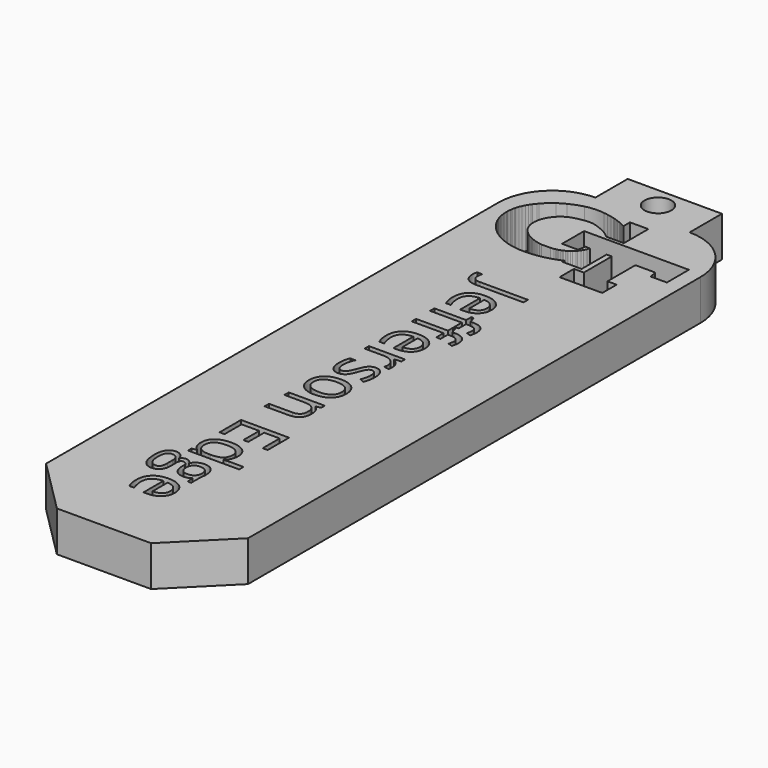
from build123d import *

# Parameters (mm, degrees)
F0_W         = 19.05
F0_H         = 63.5
F1_DEPTH     = 3.81
F3_DEPTH     = 6.35
F4_TEXT_SIZE = 6.35
F5_DEPTH     = 2.54
F6_SIZE      = 5.08
F7_R         = 5.08
F8_DEPTH     = 3.81
F9_R         = 1.27
F10_DEPTH    = 25.4


# Not quite as in the source:
# - Text() gives the source's letters only with a copy of the font that has no kerning and outlines rounded to 1/6400 em; it was checked with that copy


with BuildPart() as f1:
    # F0 (on Top) → F1 (new body)
    with BuildSketch(Plane.XY):
        with Locations((9.525, -31.75)):
            Rectangle(F0_W, F0_H)
    extrude(amount=F1_DEPTH)

    # F2 (on face) → F3 (cut)
    with BuildSketch(Plane.XY.offset(3.81)):
        with BuildLine():
            Line((9.5378421247, -2.2644413319), (9.2407390475, -2.1181011107))
            Line((9.2407390475, -2.1181011107), (9.1102886945, -2.0527776796))
            Line((9.1102886945, -2.0527776796), (8.9146168903, -1.965665957))
            Line((8.9146168903, -1.965665957), (8.6917765439, -1.8894104287))
            Line((8.6917765439, -1.8894104287), (8.4852408618, -1.8186018569))
            Line((8.4852408618, -1.8186018569), (8.3145668104, -1.7600880656))
            Line((8.3145668104, -1.7600880656), (8.1455632092, -1.7021469703))
            Line((8.1455632092, -1.7021469703), (7.8873885795, -1.6551206354))
            Line((7.8873885795, -1.6551206354), (7.4634635821, -1.5624271473))
            Line((7.4634635821, -1.5624271473), (7.1102017537, -1.5132720582))
            ThreePointArc((7.1102017537, -1.5132720582), (6.2139659935, -1.4764534117), (5.3274994716, -1.6134616453))
            ThreePointArc((5.3274994716, -1.6134616453), (4.6842584701, -1.8166701602), (4.0674582124, -2.0898187067))
            ThreePointArc((4.0674582124, -2.0898187067), (3.7122065203, -2.285641725), (3.3699632622, -2.5034029968))
            ThreePointArc((3.3699632622, -2.5034029968), (2.8715928055, -2.8986890152), (2.4355170317, -3.3617895097))
            ThreePointArc((2.4355170317, -3.3617895097), (2.3940291823, -3.4084160805), (2.3485836573, -3.4511943813))
            ThreePointArc((2.3485836573, -3.4511943813), (2.2213322779, -3.5828546335), (2.1201616619, -3.735471284))
            ThreePointArc((2.1201616619, -3.735471284), (2.0973435933, -3.7749582398), (2.0721929614, -3.8130020257))
            ThreePointArc((2.0721929614, -3.8130020257), (2.014370093, -3.8965010869), (1.9579818472, -3.9809755981))
            ThreePointArc((1.9579818472, -3.9809755981), (1.9000717817, -4.0734925924), (1.8460549181, -4.1683353484))
            ThreePointArc((1.8460549181, -4.1683353484), (1.7786496453, -4.2980206589), (1.7158541596, -4.4299997389))
            ThreePointArc((1.7158541596, -4.4299997389), (1.6653732895, -4.5386535442), (1.6130642034, -4.6464391053))
            ThreePointArc((1.6130642034, -4.6464391053), (1.5512057078, -4.8038275844), (1.5171269188, -4.9694664776))
            ThreePointArc((1.5171269188, -4.9694664776), (1.5078972179, -5.0225060098), (1.492883428, -5.0742067397))
            ThreePointArc((1.492883428, -5.0742067397), (1.4633690455, -5.183987141), (1.4506259467, -5.2969492972))
            ThreePointArc((1.4506259467, -5.2969492972), (1.4436282751, -5.3705495464), (1.4282154152, -5.4428572766))
            ThreePointArc((1.4282154152, -5.4428572766), (1.4006025542, -5.5877761483), (1.3962362427, -5.735237617))
            ThreePointArc((1.3962362427, -5.735237617), (1.3977135703, -5.794627592), (1.3962362427, -5.8540175669))
            ThreePointArc((1.3962362427, -5.8540175669), (1.3952849544, -6.0302065426), (1.4099415857, -6.2057874165))
            ThreePointArc((1.4099415857, -6.2057874165), (1.4393194847, -6.4140518173), (1.4738998143, -6.621515844))
            ThreePointArc((1.4738998143, -6.621515844), (1.5324423474, -6.8613119231), (1.6200899845, -7.0920656435))
            ThreePointArc((1.6200899845, -7.0920656435), (1.6661881926, -7.206802643), (1.7023220425, -7.3250564747))
            Line((1.7023220425, -7.3250564747), (1.805669046, -7.5137233362))
            Line((1.805669046, -7.5137233362), (1.9034598954, -7.6957228594))
            Line((1.9034598954, -7.6957228594), (1.9931015559, -7.8396927565))
            Line((1.9931015559, -7.8396927565), (2.0800267812, -7.9755131155))
            Line((2.0800267812, -7.9755131155), (2.2840281017, -8.2351164892))
            Line((2.2840281017, -8.2351164892), (2.4338501971, -8.4041468799))
            Line((2.4338501971, -8.4041468799), (2.5606225245, -8.5462853312))
            Line((2.5606225245, -8.5462853312), (2.7334939223, -8.7037906051))
            Line((2.7334939223, -8.7037906051), (2.9370982666, -8.8881868869))
            Line((2.9370982666, -8.8881868869), (3.1368609052, -9.0264836326))
            Line((3.1368609052, -9.0264836326), (3.3631285187, -9.179954417))
            Line((3.3631285187, -9.179954417), (3.5315460991, -9.2858942226))
            Line((3.5315460991, -9.2858942226), (3.6782324314, -9.3673868105))
            Line((3.6782324314, -9.3673868105), (3.9953328669, -9.5141371712))
            Line((3.9953328669, -9.5141371712), (4.220795352, -9.6064945683))
            Line((4.220795352, -9.6064945683), (4.4109444134, -9.6798380837))
            Line((4.4109444134, -9.6798380837), (4.5956601389, -9.7395991907))
            Line((4.5956601389, -9.7395991907), (4.7966749407, -9.7993602976))
            Line((4.7966749407, -9.7993602976), (4.9569434486, -9.8346732557))
            ThreePointArc((4.9569434486, -9.8346732557), (4.9706774883, -9.8382413201), (4.9841073342, -9.8428232595))
            ThreePointArc((4.9841073342, -9.8428232595), (5.081619843, -9.8720211698), (5.1824054681, -9.8862852901))
            ThreePointArc((5.1824054681, -9.8862852901), (5.1988396645, -9.8881885133), (5.2150026895, -9.891718626))
            ThreePointArc((5.2150026895, -9.891718626), (5.2809693196, -9.9053241848), (5.3481068462, -9.910733439))
            Line((5.3481068462, -9.910733439), (5.4808640853, -9.9343145266))
            Line((5.4808640853, -9.9343145266), (5.6652603671, -9.957363829))
            Line((5.6652603671, -9.957363829), (5.7766665705, -9.9727306515))
            Line((5.7766665705, -9.9727306515), (5.9360922314, -9.9880965427))
            Line((5.9360922314, -9.9880965427), (6.4451028593, -9.9880965427))
            ThreePointArc((6.4451028593, -9.9880965427), (7.3108593806, -9.9359224824), (8.1640845165, -9.7801554948))
            ThreePointArc((8.1640845165, -9.7801554948), (8.8865676974, -9.5688952176), (9.5878457651, -9.2953592539))
            Line((9.5878457651, -9.2953592539), (9.5878457651, -9.5244571567))
            Line((9.5878457651, -9.5244571567), (11.4035503939, -9.5244571567))
            Line((11.4035503939, -9.5244571567), (11.4035503939, -6.5790936351))
            Line((11.4035503939, -6.5790936351), (11.8882758543, -6.5790936351))
            Line((11.8882758543, -6.5790936351), (11.8882758543, -9.8716514185))
            Line((11.8882758543, -9.8716514185), (10.9550505877, -9.8716514185))
            Line((10.9550505877, -9.8716514185), (10.9550505877, -11.5619758144))
            Line((10.9550505877, -11.5619758144), (14.9844186381, -11.5619758144))
            Line((14.9844186381, -11.5619758144), (14.9844186381, -9.8716514185))
            Line((14.9844186381, -9.8716514185), (14.1217662022, -9.8716514185))
            Line((14.1217662022, -9.8716514185), (14.1217662022, -6.5798861906))
            Line((14.1217662022, -6.5798861906), (15.9907210618, -6.5798861906))
            Line((15.9907210618, -6.5798861906), (16.1400519139, -7.2933631585))
            Line((16.1400519139, -7.2933631585), (17.6561195403, -7.2933631585))
            Line((17.6561195403, -7.2933631585), (17.6561195403, -4.6923318878))
            Line((17.6561195403, -4.6923318878), (7.771729026, -4.6923318878))
            Line((7.771729026, -4.6923318878), (7.771729026, -7.2933631585))
            Line((7.771729026, -7.2933631585), (9.2793162912, -7.2933631585))
            Line((9.2793162912, -7.2933631585), (9.3980953097, -6.5798861906))
            Line((9.3980953097, -6.5798861906), (9.8275290802, -6.5798861906))
            Line((9.8275290802, -6.5798861906), (9.7498660907, -6.83313841))
            Line((9.7498660907, -6.83313841), (9.6219489351, -7.0935399272))
            Line((9.6219489351, -7.0935399272), (9.5214433968, -7.2488668375))
            Line((9.5214433968, -7.2488668375), (9.3524111435, -7.4727204628))
            Line((9.3524111435, -7.4727204628), (9.2838844284, -7.5458157808))
            Line((9.2838844284, -7.5458157808), (9.104157798, -7.7286572196))
            Line((9.104157798, -7.7286572196), (8.9990831912, -7.8086047433))
            Line((8.9990831912, -7.8086047433), (8.8414726779, -7.9159634188))
            Line((8.8414726779, -7.9159634188), (8.7644336745, -7.9583311453))
            Line((8.7644336745, -7.9583311453), (8.6844861507, -8.0017307773))
            Line((8.6844861507, -8.0017307773), (8.5382955149, -8.0702574924))
            Line((8.5382955149, -8.0702574924), (8.4606325254, -8.1045208499))
            Line((8.4606325254, -8.1045208499), (8.3418525755, -8.1502059475))
            Line((8.3418525755, -8.1502059475), (8.2619050518, -8.1753320992))
            Line((8.2619050518, -8.1753320992), (8.181957528, -8.2050273195))
            Line((8.181957528, -8.2050273195), (8.0974409357, -8.225585334))
            Line((8.0974409357, -8.225585334), (8.0220615491, -8.2438588142))
            Line((8.0220615491, -8.2438588142), (7.9101352021, -8.2621322945))
            Line((7.9101352021, -8.2621322945), (7.8027765267, -8.2895429805))
            Line((7.8027765267, -8.2895429805), (7.5149643235, -8.323806338))
            Line((7.5149643235, -8.323806338), (7.4121742509, -8.323806338))
            Line((7.4121742509, -8.323806338), (7.1015199646, -8.323806338))
            Line((7.1015199646, -8.323806338), (6.9416244514, -8.323806338))
            Line((6.9416244514, -8.323806338), (6.8251295015, -8.323806338))
            Line((6.8251295015, -8.323806338), (6.7923241295, -8.323806338))
            Line((6.7923241295, -8.323806338), (6.6687669605, -8.323806338))
            Line((6.6687669605, -8.323806338), (6.4426404424, -8.2954987884))
            Line((6.4426404424, -8.2954987884), (6.1632129364, -8.2341218367))
            Line((6.1632129364, -8.2341218367), (5.9193191119, -8.1662843004))
            Line((5.9193191119, -8.1662843004), (5.677041132, -8.0758333206))
            Line((5.677041132, -8.0758333206), (5.5801295675, -8.0354539678))
            Line((5.5801295675, -8.0354539678), (5.4627689533, -7.9862428829))
            Line((5.4627689533, -7.9862428829), (5.1900162362, -7.8402627259))
            Line((5.1900162362, -7.8402627259), (5.0555607304, -7.7557479963))
            Line((5.0555607304, -7.7557479963), (4.8692435957, -7.6212920249))
            Line((4.8692435957, -7.6212920249), (4.7578373924, -7.5310147367))
            Line((4.7578373924, -7.5310147367), (4.6099363826, -7.3907971382))
            Line((4.6099363826, -7.3907971382), (4.5503918082, -7.3312520981))
            Line((4.5503918082, -7.3312520981), (4.4889263809, -7.2582620196))
            Line((4.4889263809, -7.2582620196), (4.4216983952, -7.1737472899))
            ThreePointArc((4.4216983952, -7.1737472899), (4.0707252636, -6.492606789), (4.0068626404, -5.7290256955))
            ThreePointArc((4.0068626404, -5.7290256955), (4.1275399159, -5.1859398188), (4.3597090989, -4.680368118))
            ThreePointArc((4.3597090989, -4.680368118), (5.001746692, -3.9598255252), (5.8664777316, -3.5312999971))
            ThreePointArc((5.8664777316, -3.5312999971), (6.4399899486, -3.4028861901), (7.0232260041, -3.3304840326))
            ThreePointArc((7.0232260041, -3.3304840326), (7.5086797218, -3.3464679909), (7.9794181511, -3.4661598038))
            ThreePointArc((7.9794181511, -3.4661598038), (8.3595687415, -3.6141921798), (8.7353261188, -3.7730457261))
            ThreePointArc((8.7353261188, -3.7730457261), (8.9183869971, -3.8653913811), (9.0906675905, -3.9765597321))
            ThreePointArc((9.0906675905, -3.9765597321), (9.3604703513, -4.1726701979), (9.6292644739, -4.3701608665))
            Line((9.6292644739, -4.3701608665), (11.2647674978, -4.3701608665))
            Line((11.2647674978, -4.3701608665), (11.2647674978, -1.4898394002))
            Line((11.2647674978, -1.4898394002), (9.5378421247, -1.4898394002))
            Line((9.5378421247, -1.4898394002), (9.5378421247, -2.2644413319))
        make_face()
    extrude(amount=-F3_DEPTH, mode=Mode.SUBTRACT)

    # F4 (on face) → F5 (cut)
    with BuildSketch(Plane.XY.offset(3.81)):
        with Locations(Location((6.858, -15.249921875), (0, 0, -90))):
            Text('Jefferson Edge', F4_TEXT_SIZE, font='Open Sans', text_align=(TextAlign.LEFT, TextAlign.BOTTOM))
    extrude(amount=-F5_DEPTH, mode=Mode.SUBTRACT)

    # F6
    f6_edges = [f1.edges().sort_by_distance(p)[0] for p in [
        (19.05, -63.5, 1.905),
        (0, -63.5, 1.905),
    ]]
    chamfer(f6_edges, length=F6_SIZE)

    # F7
    f7_edges = [f1.edges().sort_by_distance(p)[0] for p in [
        (0, 0, 1.905),
        (19.05, 0, 1.905),
    ]]
    fillet(f7_edges, radius=F7_R)

    # F8 (add): a face of the model
    f8_faces = [f1.faces().sort_by_distance(p)[0] for p in [
        (9.525, 0, 1.905),
    ]]
    extrude(f8_faces, amount=F8_DEPTH)

    # F9 (on face) → F10 (cut)
    with BuildSketch(Plane.XY.offset(3.81)):
        with Locations((9.4615, 1.905)):
            Circle(F9_R)
    extrude(amount=-F10_DEPTH, mode=Mode.SUBTRACT)


solid = f1.part
